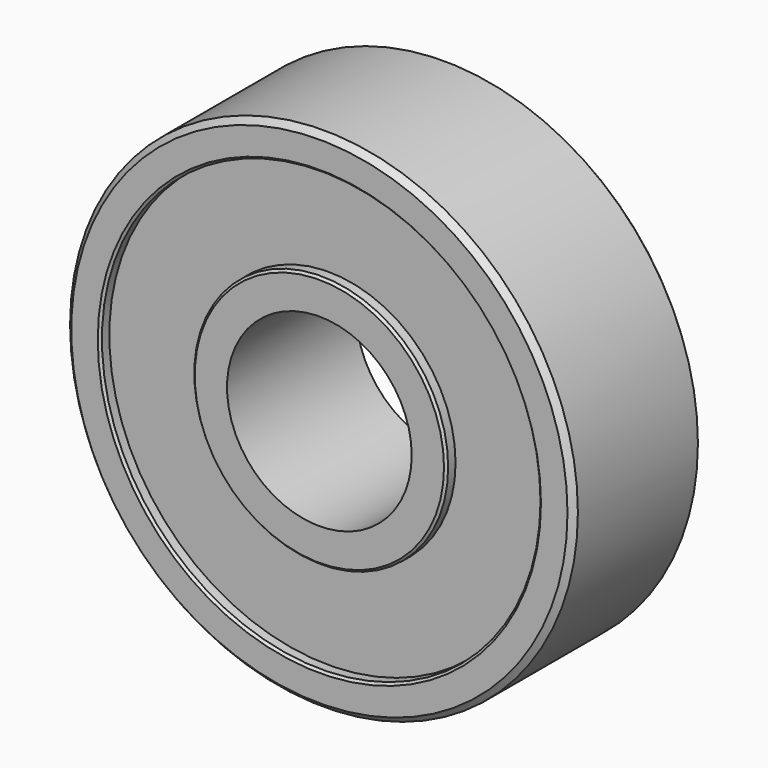
from build123d import *

# Parameters (mm, degrees)
F0_R     = 11
F0_R_2   = 4
F1_DEPTH = 3.5
F2_R     = 9.5
F2_R_2   = 5.5
F3_DEPTH = 0.5
F4_SIZE  = 0.25
F5_SIZE  = 0.1


# Not quite as in the source:
# - a pattern or mirror of a feature is missing from the dataset's text; its kind, count and spacing are read off the source's solid


with BuildPart() as f1:
    # F0 (on Front) → F1 (new body, symmetric)
    with BuildSketch(Plane.XZ):
        Circle(F0_R)
        Circle(F0_R_2, mode=Mode.SUBTRACT)
    extrude(amount=F1_DEPTH, both=True)

    # F2 (on face) → F3 (cut)
    with BuildSketch(Plane.XZ.offset(3.5)):
        Circle(F2_R)
        Circle(F2_R_2, mode=Mode.SUBTRACT)
    f3 = extrude(amount=-F3_DEPTH, mode=Mode.SUBTRACT)

    # F3_copies: F3 across plane
    add(f3.mirror(Plane.ZX), mode=Mode.SUBTRACT)

    # F4
    f4_edges = [f1.edges().sort_by_distance(p)[0] for p in [
        (-11, -3.5, 0),
        (-11, 3.5, 0),
    ]]
    chamfer(f4_edges, length=F4_SIZE)

    # F5
    f5_edges = [f1.edges().sort_by_distance(p)[0] for p in [
        (-9.5, -3.5, 0),
        (-5.5, -3.5, 0),
        (-9.5, 3.5, 0),
        (-5.5, 3.5, 0),
    ]]
    chamfer(f5_edges, length=F5_SIZE)


solid = f1.part
